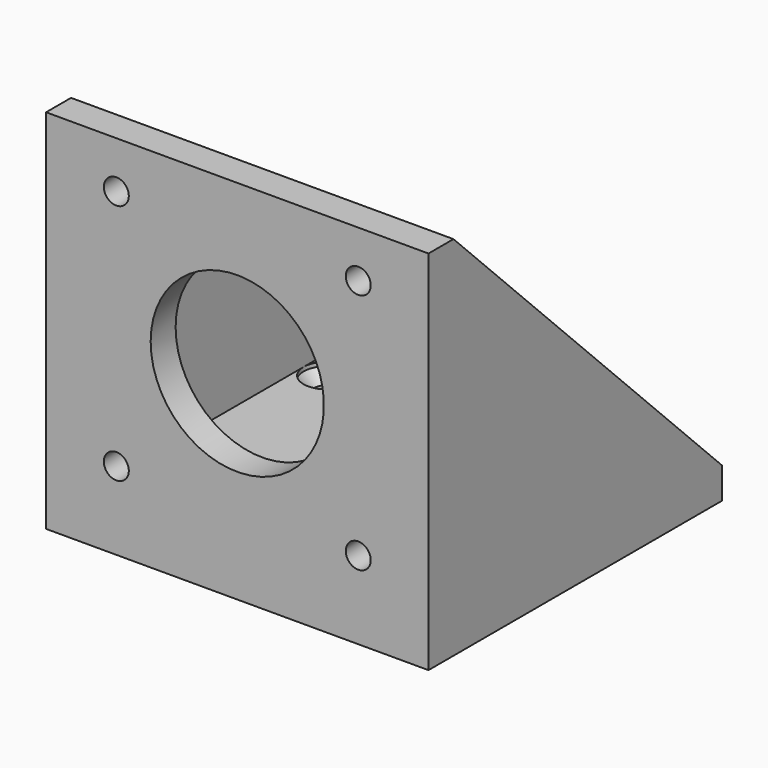
from build123d import *

# Parameters (mm, degrees)
F2_DEPTH = 24.5
F0_W     = 43
F0_H     = 43
F3_DEPTH = 21.5
F5_R     = 11.1
F5_R_2   = 1.6
F6_DEPTH = 4


# Not quite as in the source:
# - a feature of the source that left no trace in its solid (it failed there, or was rolled back) is left out


with BuildPart() as f2:
    # F1 (on Right) → F2 (new body, symmetric)
    with BuildSketch(Plane.YZ):
        Polygon((21.5, 0), (-21.5, 43), (-25.5, 43), (-25.5, -4), (21.5, -4), align=None)
    extrude(amount=F2_DEPTH, both=True)

    # F0 (on Right) → F3 (cut, symmetric)
    with BuildSketch(Plane.YZ):
        with Locations((0, 21.5)):
            Rectangle(F0_W, F0_H)
    extrude(amount=F3_DEPTH, both=True, mode=Mode.SUBTRACT)

    # F5 (on face) → F6 (cut, through all)
    with BuildSketch(Plane(origin=(0, -21.5, 0), x_dir=(-1, 0, 0), z_dir=(0, 1, 0))):
        with Locations((0, 21.5)):
            Circle(F5_R)
        with Locations((15.5, 37)):
            Circle(F5_R_2)
        with Locations((-15.5, 37)):
            Circle(F5_R_2)
        with Locations((-15.5, 6)):
            Circle(F5_R_2)
        with Locations((15.5, 6)):
            Circle(F5_R_2)
    extrude(amount=-F6_DEPTH, mode=Mode.SUBTRACT)


with BuildPart() as f7:
    # F13 (on Front) → F7 (revolve)
    with BuildSketch(Plane.XZ):
        Polygon((0, -7.6705187887), (0, 0), (-3, 0), (-3, -0.5), (-1.6, -1.9), (-1.6, -7.6705187887), align=None)
    revolve(axis=Axis((0, 0, -3.8352593944), (0, 0, 1)))


with BuildPart() as f14_1:
    # F14: copy of F7
    add(f7.part.moved(Location((0, 12, 0))))


with BuildPart() as f8_1:
    # F8: copy of F7
    add(f7.part.moved(Location((0, -12, 0))))


with BuildPart() as f9_1:
    # F9: copy of F14_1
    add(f14_1.part.moved(Location((18.5, 0, 0))))


with BuildPart() as f10_1:
    # F10: instance of F9_1
    add(f9_1.part.mirror(Plane.YZ))


with BuildPart() as f15_1:
    # F15: instance of F9_1
    add(f9_1.part.mirror(Plane.XZ))


with BuildPart() as f15_2:
    # F15: instance of F10_1
    add(f10_1.part.mirror(Plane.XZ))


with BuildPart() as f2_1:
    add(f2.part)

    # F11: cut F15_1, F8_1, F15_2, F9_1, F14_1, F10_1, F7
    add(f15_1.part, mode=Mode.SUBTRACT)
    add(f8_1.part, mode=Mode.SUBTRACT)
    add(f15_2.part, mode=Mode.SUBTRACT)
    add(f9_1.part, mode=Mode.SUBTRACT)
    add(f14_1.part, mode=Mode.SUBTRACT)
    add(f10_1.part, mode=Mode.SUBTRACT)
    add(f7.part, mode=Mode.SUBTRACT)


solid = f2_1.part
